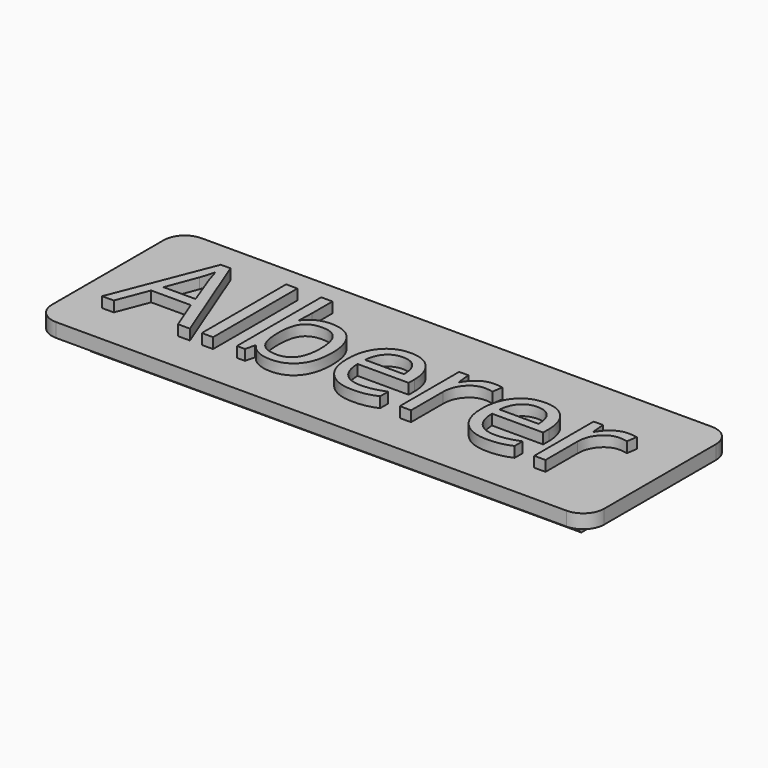
from build123d import *

# Parameters (mm, degrees)
F0_W         = 79
F0_H         = 26
F0_W_2       = 70.2
F0_H_2       = 2
F0_W_3       = 50.2
F0_W_4       = 10
F1_DEPTH     = 2
F2_DEPTH     = 5
F3_START     = -2
F3_DEPTH     = 1.3
F4_SIZE      = 1
F5_T1_DEPTH  = 20.2867319519
F5_T3_DEPTH  = 20.2867319519
F6_TEXT_SIZE = 19.8443252076
F7_DEPTH     = 1.5
F8_R         = 3


# Not quite as in the source:
# - a fillet or chamfer that OpenCascade refuses, or shapes differently, is made with other operations: its cross-section is extruded or revolved along the edge and cut away or added
# - Text() gives the source's letters only with a copy of the font that has no kerning and outlines rounded to 1/6400 em; it was checked with that copy


with BuildPart() as f1:
    # F0 (on Top) → F1 (new body)
    with BuildSketch(Plane.XY):
        Rectangle(F0_W, F0_H)
        Polygon((-35.1, -10.6), (-35.1, -8.6), (-35.1, -6.6), (-25.1, -6.6), (25.1, -6.6), (35.1, -6.6), (35.1, -8.6), (35.1, -10.6), (25.1, -10.6), (-25.1, -10.6), align=None, mode=Mode.SUBTRACT)
        Polygon((35.1, 6.6), (-35.1, 6.6), (-35.1, 8.6), (-35.1, 10.6), (35.1, 10.6), (35.1, 8.6), align=None, mode=Mode.SUBTRACT)
        with Locations((0, 7.6)):
            Rectangle(F0_W_2, F0_H_2)
        with Locations((0, 9.6)):
            Rectangle(F0_W_2, F0_H_2)
        with Locations((0, -7.6)):
            Rectangle(F0_W_3, F0_H_2)
        with Locations((0, -9.6)):
            Rectangle(F0_W_3, F0_H_2)
        with Locations((-30.1, -7.6)):
            Rectangle(F0_W_4, F0_H_2)
        with Locations((30.1, -7.6)):
            Rectangle(F0_W_4, F0_H_2)
        with Locations((-30.1, -9.6)):
            Rectangle(F0_W_4, F0_H_2)
        with Locations((30.1, -9.6)):
            Rectangle(F0_W_4, F0_H_2)
    extrude(amount=-F1_DEPTH)

    # F0 (on Top) → F2 (join)
    with BuildSketch(Plane.XY):
        with Locations((-30.1, -7.6)):
            Rectangle(F0_W_4, F0_H_2)
        with Locations((30.1, -7.6)):
            Rectangle(F0_W_4, F0_H_2)
        with Locations((0, 7.6)):
            Rectangle(F0_W_2, F0_H_2)
        with Locations((-30.1, -9.6)):
            Rectangle(F0_W_4, F0_H_2)
        with Locations((30.1, -9.6)):
            Rectangle(F0_W_4, F0_H_2)
        with Locations((0, 9.6)):
            Rectangle(F0_W_2, F0_H_2)
        with Locations((0, -7.6)):
            Rectangle(F0_W_3, F0_H_2)
    extrude(amount=-F2_DEPTH)

    # F0 (on Top) → F3 (cut)
    with BuildSketch(Plane.XY.offset(F3_START)):
        with Locations((-30.1, -9.6)):
            Rectangle(F0_W_4, F0_H_2)
        with Locations((0, -9.6)):
            Rectangle(F0_W_3, F0_H_2)
        with Locations((30.1, -9.6)):
            Rectangle(F0_W_4, F0_H_2)
        with Locations((0, 9.6)):
            Rectangle(F0_W_2, F0_H_2)
    extrude(amount=-F3_DEPTH, mode=Mode.SUBTRACT)

    # F4
    f4_edges = [f1.edges().sort_by_distance(p)[0] for p in [
        (0, 10.6, -3.3),
        (0, 6.6, -5),
        (0, 6.6, -2),
        (0, -6.6, -2),
        (0, -6.6, -5),
    ]]
    chamfer(f4_edges, length=F4_SIZE)

    # F5: chamfer of 2 on 2 edges, made by hand

    # F5_s2 → F5_t1 (cut)
    with BuildSketch(Plane.YZ.offset(-40.2433659759)):
        Polygon((-8.6, -5), (-10.6, -3), (-10.6, -5), align=None)
    extrude(amount=F5_T1_DEPTH, mode=Mode.SUBTRACT)

    # F5_s4 → F5_t3 (cut)
    with BuildSketch(Plane.YZ.offset(19.9566340241)):
        Polygon((-8.6, -5), (-10.6, -3), (-10.6, -5), align=None)
    extrude(amount=F5_T3_DEPTH, mode=Mode.SUBTRACT)

    # F6 (on face) → F7 (join)
    with BuildSketch(Plane.XY):
        with Locations((-34.6081930945, -7.1439570747)):
            Text('Alberer', F6_TEXT_SIZE, font='Open Sans', text_align=(TextAlign.LEFT, TextAlign.BOTTOM))
    extrude(amount=F7_DEPTH)

    # F8
    f8_edges = [f1.edges().sort_by_distance(p)[0] for p in [
        (39.5, 13, -1),
        (-39.5, 13, -1),
        (-39.5, -13, -1),
        (39.5, -13, -1),
    ]]
    fillet(f8_edges, radius=F8_R)


solid = f1.part
